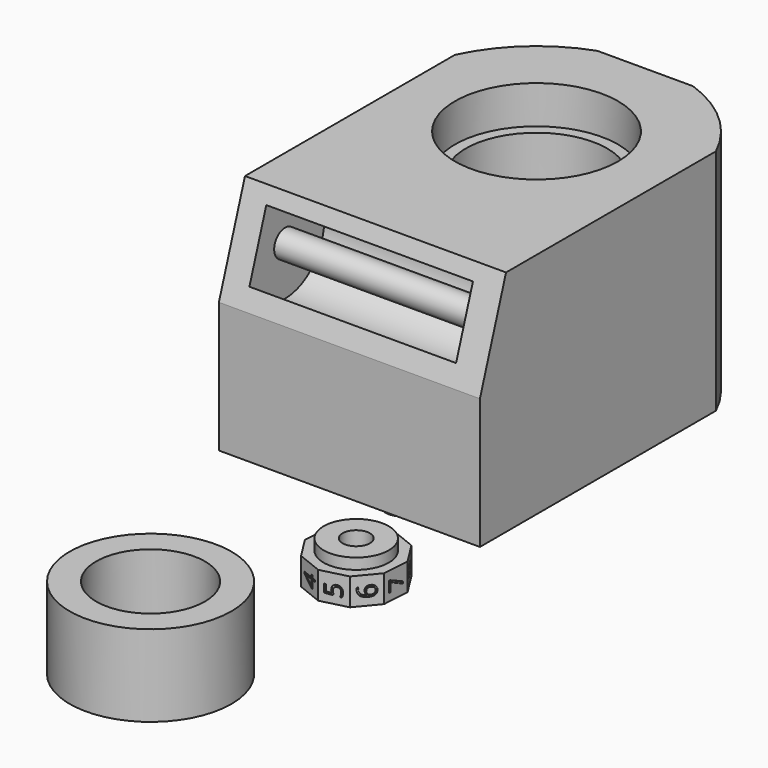
from build123d import *

# Parameters (mm, degrees)
F0_R          = 2.5
F1_DEPTH      = 5
F2_R          = 6
F2_R_2        = 2.5
F3_DEPTH      = 2
F4_TEXT_SIZE  = 4.1666666667
F5_DEPTH      = 0.2
F6_TEXT_SIZE  = 4.1666666667
F7_DEPTH      = 0.2
F8_TEXT_SIZE  = 4.1666666667
F9_DEPTH      = 0.2
F10_TEXT_SIZE = 4.1666666667
F11_DEPTH     = 0.2
F12_TEXT_SIZE = 4.1666666667
F13_DEPTH     = 0.2
F14_TEXT_SIZE = 4.1666666667
F15_DEPTH     = 0.2
F16_TEXT_SIZE = 4.1666666667
F17_DEPTH     = 0.2
F18_TEXT_SIZE = 4.1666666667
F19_DEPTH     = 0.2
F20_TEXT_SIZE = 4.1666666667
F21_DEPTH     = 0.2
F22_TEXT_SIZE = 4.1666666667
F23_DEPTH     = 0.2
F24_R         = 20
F25_DEPTH     = 14
F26_R         = 20
F26_R_2       = 13
F27_DEPTH     = 21
F28_R         = 15
F29_DEPTH     = 7
F30_R         = 2.95
F31_DEPTH     = 6.2
F33_DEPTH     = 48
F34_R         = 14.875
F34_R_2       = 10
F35_DEPTH     = 15
F36_R         = 9
F36_R_2       = 2.5
F37_DEPTH     = 38


# Not quite as in the source:
# - Text() gives the source's letters only with a copy of the font that has no kerning and outlines rounded to 1/6400 em; it was checked with that copy


with BuildPart() as f1:
    # F0 (on Top) → F1 (new body)
    with BuildSketch(Plane.XY):
        Polygon((-27.017140452, -6.0088950594), (-23.8162183671, -2.1677887336), (-23.4843636536, 2.8211863565), (-26.1483335326, 7.0524112954), (-30.7905820555, 8.9097019705), (-35.6379280707, 7.683636471), (-38.8388501556, 3.8425301451), (-39.1707048691, -1.1464449449), (-36.5067349901, -5.3776698838), (-31.8644864672, -7.2349605589), align=None)
        with Locations((-31.3275342614, 0.8373707058)):
            Circle(F0_R, mode=Mode.SUBTRACT)
    extrude(amount=F1_DEPTH)

    # F2 (on face) → F3 (join)
    with BuildSketch(Plane.XY.offset(5)):
        with Locations((-31.3275342614, 0.8373707058)):
            Circle(F2_R)
        with Locations((-31.3275342614, 0.8373707058)):
            Circle(F2_R_2, mode=Mode.SUBTRACT)
    extrude(amount=F3_DEPTH)

    # F4 (on face) → F5 (cut)
    with BuildSketch(Plane(origin=(-3.9694939045, 15.693705163, 0), x_dir=(-0.969469203, -0.2452130999, 0), z_dir=(-0.2452130999, 0.969469203, 0))):
        with Locations(Location((28.6119034471, 3.6456985527), (0, 0, -90))):
            Text('0', F4_TEXT_SIZE, font='Open Sans', text_align=(TextAlign.LEFT, TextAlign.BOTTOM))
    extrude(amount=-F5_DEPTH, mode=Mode.SUBTRACT)

    # F6 (on face) → F7 (cut)
    with BuildSketch(Plane(origin=(-24.8110566946, 20.6758815266, 0), x_dir=(-0.640184417, -0.7682212652, 0), z_dir=(-0.7682212652, 0.640184417, 0))):
        with Locations(Location((20.8071390669, 1.3786077797), (0, 0, 90))):
            Text('1', F6_TEXT_SIZE, font='Open Sans', text_align=(TextAlign.LEFT, TextAlign.BOTTOM))
    extrude(amount=-F7_DEPTH, mode=Mode.SUBTRACT)

    # F8 (on face) → F9 (cut)
    with BuildSketch(Plane(origin=(-38.9222310641, 2.5890138972, 0), x_dir=(-0.0663709427, -0.997795018, 0), z_dir=(-0.997795018, 0.0663709427, 0))):
        with Locations(Location((2.6432376405, 1.2451629934), (0, 0, 90))):
            Text('2', F8_TEXT_SIZE, font='Open Sans', text_align=(TextAlign.LEFT, TextAlign.BOTTOM))
    extrude(amount=-F9_DEPTH, mode=Mode.SUBTRACT)

    # F10 (on face) → F11 (cut)
    with BuildSketch(Plane(origin=(-28.5682420547, -17.9865021194, 0), x_dir=(0.5327939758, -0.8462449878, 0), z_dir=(-0.8462449878, -0.5327939758, 0))):
        with Locations(Location((-15.9661930444, 1.1581034267), (0, 0, 90))):
            Text('3', F10_TEXT_SIZE, font='Open Sans', text_align=(TextAlign.LEFT, TextAlign.BOTTOM))
    extrude(amount=-F11_DEPTH, mode=Mode.SUBTRACT)

    # F12 (on face) → F13 (cut)
    with BuildSketch(Plane(origin=(-6.8918929756, -17.2261027387, 0), x_dir=(0.9284497046, -0.371458135, 0), z_dir=(-0.371458135, -0.9284497046, 0))):
        with Locations(Location((-27.8585324512, 1.0578598254), (0, 0, 90))):
            Text('4', F12_TEXT_SIZE, font='Open Sans', text_align=(TextAlign.LEFT, TextAlign.BOTTOM))
    extrude(amount=-F13_DEPTH, mode=Mode.SUBTRACT)

    # F14 (on face) → F15 (cut)
    with BuildSketch(Plane(origin=(-0.1960523011, 0.7751081331, 0), x_dir=(0.969469203, 0.2452130999, 0), z_dir=(0.2452130999, -0.969469203, 0))):
        with Locations(Location((-28.7902951842, 1.0451191031), (0, 0, 90))):
            Text('5', F14_TEXT_SIZE, font='Open Sans', text_align=(TextAlign.LEFT, TextAlign.BOTTOM))
    extrude(amount=-F15_DEPTH, mode=Mode.SUBTRACT)

    # F16 (on face) → F17 (cut)
    with BuildSketch(Plane(origin=(-12.9893469911, 10.8244563221, 0), x_dir=(0.640184417, 0.7682212652, 0), z_dir=(0.7682212652, -0.640184417, 0))):
        with Locations(Location((-17.9090427289, 1.1559237008), (0, 0, 90))):
            Text('6', F16_TEXT_SIZE, font='Open Sans', text_align=(TextAlign.LEFT, TextAlign.BOTTOM))
    extrude(amount=-F17_DEPTH, mode=Mode.SUBTRACT)

    # F18 (on face) → F19 (cut)
    with BuildSketch(Plane(origin=(-23.5677445621, 1.5676701085, 0), x_dir=(0.0663709427, 0.997795018, 0), z_dir=(0.997795018, -0.0663709427, 0))):
        with Locations(Location((0.2514715589, 1.2121952755), (0, 0, 90))):
            Text('7', F18_TEXT_SIZE, font='Open Sans', text_align=(TextAlign.LEFT, TextAlign.BOTTOM))
    extrude(amount=-F19_DEPTH, mode=Mode.SUBTRACT)

    # F20 (on face) → F21 (cut)
    with BuildSketch(Plane(origin=(-15.5458707181, -9.7876458791, 0), x_dir=(-0.5327939758, 0.8462449878, 0), z_dir=(0.8462449878, 0.5327939758, 0))):
        with Locations(Location((18.9492461354, 1.181016458), (0, 0, 90))):
            Text('8', F20_TEXT_SIZE, font='Open Sans', text_align=(TextAlign.LEFT, TextAlign.BOTTOM))
    extrude(amount=-F21_DEPTH, mode=Mode.SUBTRACT)

    # F22 (on face) → F23 (cut)
    with BuildSketch(Plane(origin=(-1.1757400409, -2.9387308844, 0), x_dir=(-0.9284497046, 0.371458135, 0), z_dir=(0.371458135, 0.9284497046, 0))):
        with Locations(Location((30.7762525978, 1.1026628106), (0, 0, 90))):
            Text('9', F22_TEXT_SIZE, font='Open Sans', text_align=(TextAlign.LEFT, TextAlign.BOTTOM))
    extrude(amount=-F23_DEPTH, mode=Mode.SUBTRACT)


with BuildPart() as f25:
    # F24 (on Top) → F25 (new body)
    with BuildSketch(Plane.XY):
        with BuildLine():
            Line((-39.3768328937, 88.3187037259), (-56.9552287249, 88.3187037259))
            ThreePointArc((-56.9552287249, 88.3187037259), (-65.9464721255, 82.9682814975), (-72.1660308093, 74.5548062531))
            Line((-72.1660308093, 74.5548062531), (-72.1660308093, 20.3187037259))
            Line((-72.1660308093, 20.3187037259), (-24.1660308093, 20.3187037259))
            Line((-24.1660308093, 20.3187037259), (-24.1660308093, 74.5548062531))
            ThreePointArc((-24.1660308093, 74.5548062531), (-30.3855894931, 82.9682814975), (-39.3768328937, 88.3187037259))
        make_face()
        with Locations((-48.1660308093, 63.3187037259)):
            Circle(F24_R, mode=Mode.SUBTRACT)
    extrude(amount=F25_DEPTH)

    # F26 (on face) → F27 (join)
    with BuildSketch(Plane.XY.offset(14)):
        with BuildLine():
            ThreePointArc((-56.9552287249, 88.3187037259), (-65.9464721255, 82.9682814975), (-72.1660308093, 74.5548062531))
            Line((-72.1660308093, 74.5548062531), (-72.1660308093, 20.3187037259))
            Line((-72.1660308093, 20.3187037259), (-24.1660308093, 20.3187037259))
            Line((-24.1660308093, 20.3187037259), (-24.1660308093, 74.5548062531))
            ThreePointArc((-24.1660308093, 74.5548062531), (-30.3855894931, 82.9682814975), (-39.3768328937, 88.3187037259))
            Line((-39.3768328937, 88.3187037259), (-56.9552287249, 88.3187037259))
        make_face()
        with Locations((-48.1660308093, 63.3187037259)):
            Circle(F26_R, mode=Mode.SUBTRACT)
        with Locations((-48.1660308093, 63.3187037259)):
            Circle(F26_R)
        with Locations((-48.1660308093, 63.3187037259)):
            Circle(F26_R_2, mode=Mode.SUBTRACT)
    extrude(amount=F27_DEPTH)

    # F28 (on face) → F29 (join)
    with BuildSketch(Plane.XY.offset(35)):
        with BuildLine():
            Line((-39.3768328937, 88.3187037259), (-56.9552287249, 88.3187037259))
            ThreePointArc((-56.9552287249, 88.3187037259), (-65.9464721255, 82.9682814975), (-72.1660308093, 74.5548062531))
            Line((-72.1660308093, 74.5548062531), (-72.1660308093, 20.3187037259))
            Line((-72.1660308093, 20.3187037259), (-24.1660308093, 20.3187037259))
            Line((-24.1660308093, 20.3187037259), (-24.1660308093, 74.5548062531))
            ThreePointArc((-24.1660308093, 74.5548062531), (-30.3855894931, 82.9682814975), (-39.3768328937, 88.3187037259))
        make_face()
        with Locations((-48.1660308093, 63.3187037259)):
            Circle(F28_R, mode=Mode.SUBTRACT)
    extrude(amount=F29_DEPTH)

    # F30 (on face) → F31 (join)
    with BuildSketch(Plane(origin=(0, 0, 0), x_dir=(1, 0, 0), z_dir=(0, 0, -1))):
        with Locations((-48.1660308093, -32.3187037259)):
            Circle(F30_R)
    extrude(amount=F31_DEPTH)

    # F32 (on face) → F33 (cut, through all)
    with BuildSketch(Plane.YZ.offset(-24.1660308093)):
        Polygon((26.3187037259, 42), (20.3187037259, 42), (20.3187037259, 24), align=None)
    extrude(amount=-F33_DEPTH, mode=Mode.SUBTRACT)


with BuildPart() as f35:
    # F34 (on Top) → F35 (new body)
    with BuildSketch(Plane.XY):
        with Locations((-36.3977178931, -40.0992147624)):
            Circle(F34_R)
        with Locations((-36.3977178931, -40.0992147624)):
            Circle(F34_R_2, mode=Mode.SUBTRACT)
    extrude(amount=F35_DEPTH)


with BuildPart() as f37:
    # F36 (on Right) → F37 (new body)
    with BuildSketch(Plane.YZ):
        with Locations((42.2904267907, 66.2897825241)):
            Circle(F36_R)
        with Locations((42.2904267907, 66.2897825241)):
            Circle(F36_R_2, mode=Mode.SUBTRACT)
    extrude(amount=F37_DEPTH)


with BuildPart() as f37_1:
    # F38: moved
    add(f37.part.moved(Location((-67.5, -12.6, -35))))


with BuildPart() as f25_1:
    add(f25.part)

    # F39: cut F37
    add(f37_1.part, mode=Mode.SUBTRACT)


solid = Compound([f1.part, f35.part, f25_1.part])
